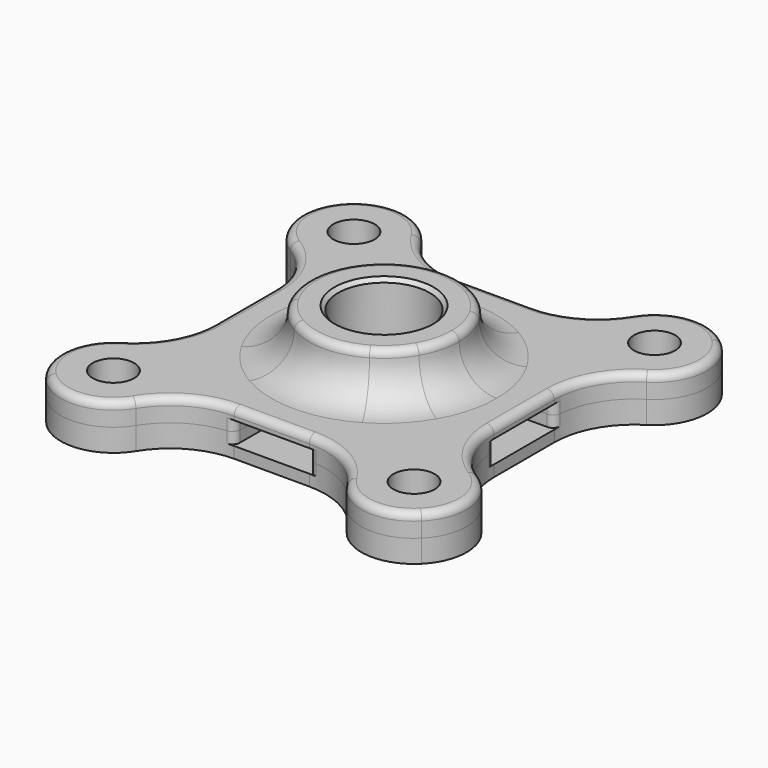
from build123d import *

# Parameters (mm, degrees)
F0_R           = 2.75
F0_R_2         = 9.25
F0_R_3         = 6.1
F1_DEPTH       = 3
F2_DEPTH       = 9
F3_DEPTH       = 1.5
F0_R_4         = 5
F4_DEPTH       = 3
F5_DEPTH       = 1.5
F6_SIZE        = 0.5
F7_R           = 5
F8_F1_R        = 0.9999
F8_F2_R        = 1
F8_2_T4_ANGLE  = 58.6491681138
F8_2_T10_ANGLE = 58.6491681138
F8_2_T16_ANGLE = 58.6491681138
F8_2_T22_ANGLE = 58.6491681138
F8_2_T25_DEPTH = 3.8925933322


# Not quite as in the source:
# - a fillet or chamfer that OpenCascade refuses, or shapes differently, is made with other operations: its cross-section is extruded or revolved along the edge and cut away or added
# - a fillet or chamfer is up to 0.001 mm smaller than in the source, because OpenCascade refuses the exact size
# - a feature names something its author has since deleted; it is built from what else it names


with BuildPart() as f1:
    # F0 (on Top) → F1 (new body)
    with BuildSketch(Plane.XY):
        with BuildLine():
            ThreePointArc((8.6602540378, 5), (9.6592582629, 2.588190451), (10, 0))
            ThreePointArc((10, 0), (9.6592582629, -2.588190451), (8.6602540378, -5))
            Line((8.6602540378, -5), (18.6602540378, -5))
            Line((18.6602540378, -5), (18.6602540378, 0))
            Line((18.6602540378, 0), (18.6602540378, 5))
            Line((18.6602540378, 5), (8.6602540378, 5))
        make_face()
        with BuildLine():
            ThreePointArc((5, 8.6602540378), (7.0710678119, 7.0710678119), (8.6602540378, 5))
            Line((8.6602540378, 5), (18.6602540378, 5))
            ThreePointArc((18.6602540378, 5), (20.0033649329, 10.1797503972), (23.6942299332, 14.0541892731))
            ThreePointArc((23.6942299332, 14.0541892731), (26.9539832777, 19.1986782332), (24.9497474683, 24.9497474683))
            ThreePointArc((24.9497474683, 24.9497474683), (19.1986782332, 26.9539832777), (14.0541892731, 23.6942299332))
            ThreePointArc((14.0541892731, 23.6942299332), (10.1797503972, 20.0033649329), (5, 18.6602540378))
            Line((5, 18.6602540378), (5, 8.6602540378))
        make_face()
        with Locations((20, 20)):
            Circle(F0_R, mode=Mode.SUBTRACT)
        with BuildLine():
            Line((18.6602540378, -5), (8.6602540378, -5))
            ThreePointArc((8.6602540378, -5), (7.0710678119, -7.0710678119), (5, -8.6602540378))
            Line((5, -8.6602540378), (5, -18.6602540378))
            ThreePointArc((5, -18.6602540378), (10.1797503972, -20.0033649329), (14.0541892731, -23.6942299332))
            ThreePointArc((14.0541892731, -23.6942299332), (19.1986782332, -26.9539832777), (24.9497474683, -24.9497474683))
            ThreePointArc((24.9497474683, -24.9497474683), (26.9539832777, -19.1986782332), (23.6942299332, -14.0541892731))
            ThreePointArc((23.6942299332, -14.0541892731), (20.0033649329, -10.1797503972), (18.6602540378, -5))
        make_face()
        with Locations((20, -20)):
            Circle(F0_R, mode=Mode.SUBTRACT)
        with BuildLine():
            ThreePointArc((-8.6602540378, 5), (-7.0710678119, 7.0710678119), (-5, 8.6602540378))
            Line((-5, 8.6602540378), (-5, 18.6602540378))
            ThreePointArc((-5, 18.6602540378), (-10.1797503972, 20.0033649329), (-14.0541892731, 23.6942299332))
            ThreePointArc((-14.0541892731, 23.6942299332), (-19.1986782332, 26.9539832777), (-24.9497474683, 24.9497474683))
            ThreePointArc((-24.9497474683, 24.9497474683), (-26.9539832777, 19.1986782332), (-23.6942299332, 14.0541892731))
            ThreePointArc((-23.6942299332, 14.0541892731), (-20.0033649329, 10.1797503972), (-18.6602540378, 5))
            Line((-18.6602540378, 5), (-8.6602540378, 5))
        make_face()
        with Locations((-20, 20)):
            Circle(F0_R, mode=Mode.SUBTRACT)
        with BuildLine():
            ThreePointArc((8.6602540378, -5), (9.6592582629, -2.588190451), (10, 0))
            ThreePointArc((10, 0), (9.6592582629, 2.588190451), (8.6602540378, 5))
            ThreePointArc((8.6602540378, 5), (7.0710678119, 7.0710678119), (5, 8.6602540378))
            ThreePointArc((5, 8.6602540378), (0, 10), (-5, 8.6602540378))
            ThreePointArc((-5, 8.6602540378), (-7.0710678119, 7.0710678119), (-8.6602540378, 5))
            ThreePointArc((-8.6602540378, 5), (-10, 0), (-8.6602540378, -5))
            ThreePointArc((-8.6602540378, -5), (-7.0710678119, -7.0710678119), (-5, -8.6602540378))
            ThreePointArc((-5, -8.6602540378), (0, -10), (5, -8.6602540378))
            ThreePointArc((5, -8.6602540378), (7.0710678119, -7.0710678119), (8.6602540378, -5))
        make_face()
        Circle(F0_R_2, mode=Mode.SUBTRACT)
        with BuildLine():
            Line((-5, -18.6602540378), (-5, -8.6602540378))
            ThreePointArc((-5, -8.6602540378), (-7.0710678119, -7.0710678119), (-8.6602540378, -5))
            Line((-8.6602540378, -5), (-18.6602540378, -5))
            ThreePointArc((-18.6602540378, -5), (-20.0033649329, -10.1797503972), (-23.6942299332, -14.0541892731))
            ThreePointArc((-23.6942299332, -14.0541892731), (-26.9539832777, -19.1986782332), (-24.9497474683, -24.9497474683))
            ThreePointArc((-24.9497474683, -24.9497474683), (-19.1986782332, -26.9539832777), (-14.0541892731, -23.6942299332))
            ThreePointArc((-14.0541892731, -23.6942299332), (-10.1797503972, -20.0033649329), (-5, -18.6602540378))
        make_face()
        with Locations((-20, -20)):
            Circle(F0_R, mode=Mode.SUBTRACT)
        with BuildLine():
            Line((5, -18.6602540378), (5, -8.6602540378))
            ThreePointArc((5, -8.6602540378), (0, -10), (-5, -8.6602540378))
            Line((-5, -8.6602540378), (-5, -18.6602540378))
            Line((-5, -18.6602540378), (0, -18.6602540378))
            Line((0, -18.6602540378), (5, -18.6602540378))
        make_face()
        Circle(F0_R_2)
        Circle(F0_R_3, mode=Mode.SUBTRACT)
        with BuildLine():
            ThreePointArc((-8.6602540378, -5), (-10, 0), (-8.6602540378, 5))
            Line((-8.6602540378, 5), (-18.6602540378, 5))
            Line((-18.6602540378, 5), (-18.6602540378, 0))
            Line((-18.6602540378, 0), (-18.6602540378, -5))
            Line((-18.6602540378, -5), (-8.6602540378, -5))
        make_face()
        with BuildLine():
            ThreePointArc((-5, 8.6602540378), (0, 10), (5, 8.6602540378))
            Line((5, 8.6602540378), (5, 18.6602540378))
            Line((5, 18.6602540378), (0, 18.6602540378))
            Line((0, 18.6602540378), (-5, 18.6602540378))
            Line((-5, 18.6602540378), (-5, 8.6602540378))
        make_face()
    extrude(amount=F1_DEPTH)

    # F0 (on Top) → F2 (join)
    with BuildSketch(Plane.XY):
        with BuildLine():
            ThreePointArc((8.6602540378, -5), (9.6592582629, -2.588190451), (10, 0))
            ThreePointArc((10, 0), (9.6592582629, 2.588190451), (8.6602540378, 5))
            ThreePointArc((8.6602540378, 5), (7.0710678119, 7.0710678119), (5, 8.6602540378))
            ThreePointArc((5, 8.6602540378), (0, 10), (-5, 8.6602540378))
            ThreePointArc((-5, 8.6602540378), (-7.0710678119, 7.0710678119), (-8.6602540378, 5))
            ThreePointArc((-8.6602540378, 5), (-10, 0), (-8.6602540378, -5))
            ThreePointArc((-8.6602540378, -5), (-7.0710678119, -7.0710678119), (-5, -8.6602540378))
            ThreePointArc((-5, -8.6602540378), (0, -10), (5, -8.6602540378))
            ThreePointArc((5, -8.6602540378), (7.0710678119, -7.0710678119), (8.6602540378, -5))
        make_face()
        Circle(F0_R_2, mode=Mode.SUBTRACT)
        Circle(F0_R_2)
        Circle(F0_R_3, mode=Mode.SUBTRACT)
    extrude(amount=F2_DEPTH)

    # F0 (on Top) → F3 (cut)
    with BuildSketch(Plane.XY):
        with BuildLine():
            ThreePointArc((8.6602540378, -5), (9.6592582629, -2.588190451), (10, 0))
            ThreePointArc((10, 0), (9.6592582629, 2.588190451), (8.6602540378, 5))
            ThreePointArc((8.6602540378, 5), (7.0710678119, 7.0710678119), (5, 8.6602540378))
            ThreePointArc((5, 8.6602540378), (0, 10), (-5, 8.6602540378))
            ThreePointArc((-5, 8.6602540378), (-7.0710678119, 7.0710678119), (-8.6602540378, 5))
            ThreePointArc((-8.6602540378, 5), (-10, 0), (-8.6602540378, -5))
            ThreePointArc((-8.6602540378, -5), (-7.0710678119, -7.0710678119), (-5, -8.6602540378))
            ThreePointArc((-5, -8.6602540378), (0, -10), (5, -8.6602540378))
            ThreePointArc((5, -8.6602540378), (7.0710678119, -7.0710678119), (8.6602540378, -5))
        make_face()
        Circle(F0_R_2, mode=Mode.SUBTRACT)
        Circle(F0_R_2)
        Circle(F0_R_3, mode=Mode.SUBTRACT)
        with BuildLine():
            Line((5, -18.6602540378), (5, -8.6602540378))
            ThreePointArc((5, -8.6602540378), (0, -10), (-5, -8.6602540378))
            Line((-5, -8.6602540378), (-5, -18.6602540378))
            Line((-5, -18.6602540378), (0, -18.6602540378))
            Line((0, -18.6602540378), (5, -18.6602540378))
        make_face()
        with BuildLine():
            ThreePointArc((-8.6602540378, -5), (-10, 0), (-8.6602540378, 5))
            Line((-8.6602540378, 5), (-18.6602540378, 5))
            Line((-18.6602540378, 5), (-18.6602540378, 0))
            Line((-18.6602540378, 0), (-18.6602540378, -5))
            Line((-18.6602540378, -5), (-8.6602540378, -5))
        make_face()
        with BuildLine():
            ThreePointArc((8.6602540378, 5), (9.6592582629, 2.588190451), (10, 0))
            ThreePointArc((10, 0), (9.6592582629, -2.588190451), (8.6602540378, -5))
            Line((8.6602540378, -5), (18.6602540378, -5))
            Line((18.6602540378, -5), (18.6602540378, 0))
            Line((18.6602540378, 0), (18.6602540378, 5))
            Line((18.6602540378, 5), (8.6602540378, 5))
        make_face()
        with BuildLine():
            ThreePointArc((-5, 8.6602540378), (0, 10), (5, 8.6602540378))
            Line((5, 8.6602540378), (5, 18.6602540378))
            Line((5, 18.6602540378), (0, 18.6602540378))
            Line((0, 18.6602540378), (-5, 18.6602540378))
            Line((-5, 18.6602540378), (-5, 8.6602540378))
        make_face()
    extrude(amount=F3_DEPTH, mode=Mode.SUBTRACT)

    # F6
    f6_edges = [f1.edges().sort_by_distance(p)[0] for p in [
        (-6.1, 0, 9),
    ]]
    chamfer(f6_edges, length=F6_SIZE)

    # F7
    f7_edges = [f1.edges().sort_by_distance(p)[0] for p in [
        (-8.660254, 5, 3),
    ]]
    fillet(f7_edges, radius=F7_R)

    # F8: fillet of radius 1 on 33 edges, made by hand

    # F8_f1 (radius 1 in the source; OpenCascade refuses exactly that, so slightly less here)
    f8_f1_edges = [f1.edges().sort_by_distance(p)[0] for p in [
        (18.6602540378, -5, 0.75),
        (18.6602540378, 5, 0.75),
        (5, 18.6602540378, 0.75),
        (-5, 18.6602540378, 0.75),
        (-18.6602540378, 5, 0.75),
        (-18.6602540378, -5, 0.75),
        (-5, -18.6602540378, 0.75),
        (5, -18.6602540378, 0.75),
        (-8.6602540378, 5, 9),
    ]]
    fillet(f8_f1_edges, radius=F8_F1_R)

    # F8_f2
    f8_f2_edges = [f1.edges().sort_by_distance(p)[0] for p in [
        (24.9497474683, 24.9497474683, 3),
        (-24.9497474683, 24.9497474683, 3),
        (-24.9497474683, -24.9497474683, 3),
        (24.9497474683, -24.9497474683, 3),
        (18.6602540378, 0, 3),
        (0, 18.6602540378, 3),
        (-18.6602540378, 0, 3),
        (0, -18.6602540378, 3),
        (20.0033649329, -10.1797503972, 3),
        (20.0033649329, 10.1797503972, 3),
        (10.1797503972, -20.0033649329, 3),
        (10.1797503972, 20.0033649329, 3),
        (-10.1797503972, -20.0033649329, 3),
        (-10.1797503972, 20.0033649329, 3),
        (-20.0033649329, -10.1797503972, 3),
        (-20.0033649329, 10.1797503972, 3),
    ]]
    fillet(f8_f2_edges, radius=F8_F2_R)


with BuildPart() as f4:
    # F0 (on Top) → F4 (new body)
    with BuildSketch(Plane.XY):
        with BuildLine():
            Line((-5, -18.6602540378), (-5, -8.6602540378))
            ThreePointArc((-5, -8.6602540378), (-7.0710678119, -7.0710678119), (-8.6602540378, -5))
            Line((-8.6602540378, -5), (-18.6602540378, -5))
            ThreePointArc((-18.6602540378, -5), (-20.0033649329, -10.1797503972), (-23.6942299332, -14.0541892731))
            ThreePointArc((-23.6942299332, -14.0541892731), (-26.9539832777, -19.1986782332), (-24.9497474683, -24.9497474683))
            ThreePointArc((-24.9497474683, -24.9497474683), (-19.1986782332, -26.9539832777), (-14.0541892731, -23.6942299332))
            ThreePointArc((-14.0541892731, -23.6942299332), (-10.1797503972, -20.0033649329), (-5, -18.6602540378))
        make_face()
        with Locations((-20, -20)):
            Circle(F0_R, mode=Mode.SUBTRACT)
        with BuildLine():
            Line((5, -18.6602540378), (5, -8.6602540378))
            ThreePointArc((5, -8.6602540378), (0, -10), (-5, -8.6602540378))
            Line((-5, -8.6602540378), (-5, -18.6602540378))
            Line((-5, -18.6602540378), (0, -18.6602540378))
            Line((0, -18.6602540378), (5, -18.6602540378))
        make_face()
        with BuildLine():
            Line((18.6602540378, -5), (8.6602540378, -5))
            ThreePointArc((8.6602540378, -5), (7.0710678119, -7.0710678119), (5, -8.6602540378))
            Line((5, -8.6602540378), (5, -18.6602540378))
            ThreePointArc((5, -18.6602540378), (10.1797503972, -20.0033649329), (14.0541892731, -23.6942299332))
            ThreePointArc((14.0541892731, -23.6942299332), (19.1986782332, -26.9539832777), (24.9497474683, -24.9497474683))
            ThreePointArc((24.9497474683, -24.9497474683), (26.9539832777, -19.1986782332), (23.6942299332, -14.0541892731))
            ThreePointArc((23.6942299332, -14.0541892731), (20.0033649329, -10.1797503972), (18.6602540378, -5))
        make_face()
        with Locations((20, -20)):
            Circle(F0_R, mode=Mode.SUBTRACT)
        with BuildLine():
            ThreePointArc((8.6602540378, 5), (9.6592582629, 2.588190451), (10, 0))
            ThreePointArc((10, 0), (9.6592582629, -2.588190451), (8.6602540378, -5))
            Line((8.6602540378, -5), (18.6602540378, -5))
            Line((18.6602540378, -5), (18.6602540378, 0))
            Line((18.6602540378, 0), (18.6602540378, 5))
            Line((18.6602540378, 5), (8.6602540378, 5))
        make_face()
        with BuildLine():
            ThreePointArc((5, 8.6602540378), (7.0710678119, 7.0710678119), (8.6602540378, 5))
            Line((8.6602540378, 5), (18.6602540378, 5))
            ThreePointArc((18.6602540378, 5), (20.0033649329, 10.1797503972), (23.6942299332, 14.0541892731))
            ThreePointArc((23.6942299332, 14.0541892731), (26.9539832777, 19.1986782332), (24.9497474683, 24.9497474683))
            ThreePointArc((24.9497474683, 24.9497474683), (19.1986782332, 26.9539832777), (14.0541892731, 23.6942299332))
            ThreePointArc((14.0541892731, 23.6942299332), (10.1797503972, 20.0033649329), (5, 18.6602540378))
            Line((5, 18.6602540378), (5, 8.6602540378))
        make_face()
        with Locations((20, 20)):
            Circle(F0_R, mode=Mode.SUBTRACT)
        with BuildLine():
            ThreePointArc((-5, 8.6602540378), (0, 10), (5, 8.6602540378))
            Line((5, 8.6602540378), (5, 18.6602540378))
            Line((5, 18.6602540378), (0, 18.6602540378))
            Line((0, 18.6602540378), (-5, 18.6602540378))
            Line((-5, 18.6602540378), (-5, 8.6602540378))
        make_face()
        with BuildLine():
            ThreePointArc((-8.6602540378, 5), (-7.0710678119, 7.0710678119), (-5, 8.6602540378))
            Line((-5, 8.6602540378), (-5, 18.6602540378))
            ThreePointArc((-5, 18.6602540378), (-10.1797503972, 20.0033649329), (-14.0541892731, 23.6942299332))
            ThreePointArc((-14.0541892731, 23.6942299332), (-19.1986782332, 26.9539832777), (-24.9497474683, 24.9497474683))
            ThreePointArc((-24.9497474683, 24.9497474683), (-26.9539832777, 19.1986782332), (-23.6942299332, 14.0541892731))
            ThreePointArc((-23.6942299332, 14.0541892731), (-20.0033649329, 10.1797503972), (-18.6602540378, 5))
            Line((-18.6602540378, 5), (-8.6602540378, 5))
        make_face()
        with Locations((-20, 20)):
            Circle(F0_R, mode=Mode.SUBTRACT)
        with BuildLine():
            ThreePointArc((-8.6602540378, -5), (-10, 0), (-8.6602540378, 5))
            Line((-8.6602540378, 5), (-18.6602540378, 5))
            Line((-18.6602540378, 5), (-18.6602540378, 0))
            Line((-18.6602540378, 0), (-18.6602540378, -5))
            Line((-18.6602540378, -5), (-8.6602540378, -5))
        make_face()
        with BuildLine():
            ThreePointArc((8.6602540378, -5), (9.6592582629, -2.588190451), (10, 0))
            ThreePointArc((10, 0), (9.6592582629, 2.588190451), (8.6602540378, 5))
            ThreePointArc((8.6602540378, 5), (7.0710678119, 7.0710678119), (5, 8.6602540378))
            ThreePointArc((5, 8.6602540378), (0, 10), (-5, 8.6602540378))
            ThreePointArc((-5, 8.6602540378), (-7.0710678119, 7.0710678119), (-8.6602540378, 5))
            ThreePointArc((-8.6602540378, 5), (-10, 0), (-8.6602540378, -5))
            ThreePointArc((-8.6602540378, -5), (-7.0710678119, -7.0710678119), (-5, -8.6602540378))
            ThreePointArc((-5, -8.6602540378), (0, -10), (5, -8.6602540378))
            ThreePointArc((5, -8.6602540378), (7.0710678119, -7.0710678119), (8.6602540378, -5))
        make_face()
        Circle(F0_R_2, mode=Mode.SUBTRACT)
        Circle(F0_R_2)
        Circle(F0_R_3, mode=Mode.SUBTRACT)
        Circle(F0_R_3)
        Circle(F0_R_4, mode=Mode.SUBTRACT)
        Circle(F0_R_4)
    extrude(amount=-F4_DEPTH)

    # F0 (on Top) → F5 (cut)
    with BuildSketch(Plane.XY):
        with BuildLine():
            ThreePointArc((-8.6602540378, -5), (-10, 0), (-8.6602540378, 5))
            Line((-8.6602540378, 5), (-18.6602540378, 5))
            Line((-18.6602540378, 5), (-18.6602540378, 0))
            Line((-18.6602540378, 0), (-18.6602540378, -5))
            Line((-18.6602540378, -5), (-8.6602540378, -5))
        make_face()
        with BuildLine():
            ThreePointArc((8.6602540378, -5), (9.6592582629, -2.588190451), (10, 0))
            ThreePointArc((10, 0), (9.6592582629, 2.588190451), (8.6602540378, 5))
            ThreePointArc((8.6602540378, 5), (7.0710678119, 7.0710678119), (5, 8.6602540378))
            ThreePointArc((5, 8.6602540378), (0, 10), (-5, 8.6602540378))
            ThreePointArc((-5, 8.6602540378), (-7.0710678119, 7.0710678119), (-8.6602540378, 5))
            ThreePointArc((-8.6602540378, 5), (-10, 0), (-8.6602540378, -5))
            ThreePointArc((-8.6602540378, -5), (-7.0710678119, -7.0710678119), (-5, -8.6602540378))
            ThreePointArc((-5, -8.6602540378), (0, -10), (5, -8.6602540378))
            ThreePointArc((5, -8.6602540378), (7.0710678119, -7.0710678119), (8.6602540378, -5))
        make_face()
        Circle(F0_R_2, mode=Mode.SUBTRACT)
        with BuildLine():
            ThreePointArc((-5, 8.6602540378), (0, 10), (5, 8.6602540378))
            Line((5, 8.6602540378), (5, 18.6602540378))
            Line((5, 18.6602540378), (0, 18.6602540378))
            Line((0, 18.6602540378), (-5, 18.6602540378))
            Line((-5, 18.6602540378), (-5, 8.6602540378))
        make_face()
        with BuildLine():
            ThreePointArc((8.6602540378, 5), (9.6592582629, 2.588190451), (10, 0))
            ThreePointArc((10, 0), (9.6592582629, -2.588190451), (8.6602540378, -5))
            Line((8.6602540378, -5), (18.6602540378, -5))
            Line((18.6602540378, -5), (18.6602540378, 0))
            Line((18.6602540378, 0), (18.6602540378, 5))
            Line((18.6602540378, 5), (8.6602540378, 5))
        make_face()
        with BuildLine():
            Line((5, -18.6602540378), (5, -8.6602540378))
            ThreePointArc((5, -8.6602540378), (0, -10), (-5, -8.6602540378))
            Line((-5, -8.6602540378), (-5, -18.6602540378))
            Line((-5, -18.6602540378), (0, -18.6602540378))
            Line((0, -18.6602540378), (5, -18.6602540378))
        make_face()
    extrude(amount=-F5_DEPTH, mode=Mode.SUBTRACT)

    # F8#2: fillet of radius 1 on 20 edges, made by hand


with BuildPart() as f8_2_tool2:
    # F8_2_s3 → F8_2_t4 (revolve)
    with BuildSketch(Plane(origin=(0, 0, 0), x_dir=(0, 0, 1), z_dir=(0.9628077651, 0.2701873563, 0))):
        with BuildLine():
            ThreePointArc((-1.5, -9), (-1.2071067812, -9.7071067812), (-0.5, -10))
            Line((-0.5, -10), (-1.5, -10))
            Line((-1.5, -10), (-1.5, -9))
        make_face()
    revolve(axis=Axis((0, 0, -1.5), (0, 0, 1)), revolution_arc=F8_2_T4_ANGLE)

    split(bisect_by=Plane.YZ.offset(-5), keep=Keep.BOTTOM)

    split(bisect_by=Plane.XZ.offset(-5), keep=Keep.BOTTOM)


with BuildPart() as f4_1:
    add(f4.part)

    # F8_2_t1: union F8_2_tool2
    add(f8_2_tool2.part)


with BuildPart() as f8_2_tool8:
    # F8_2_s9 → F8_2_t10 (revolve)
    with BuildSketch(Plane(origin=(0, 0, 0), x_dir=(0, 0, 1), z_dir=(-0.2701873563, 0.9628077651, 0))):
        with BuildLine():
            ThreePointArc((-0.5, -10), (-1.2071067812, -9.7071067812), (-1.5, -9))
            Line((-1.5, -9), (-1.5, -10))
            Line((-1.5, -10), (-0.5, -10))
        make_face()
    revolve(axis=Axis((0, 0, -1.5), (0, 0, 1)), revolution_arc=F8_2_T10_ANGLE)

    split(bisect_by=Plane.YZ.offset(-5), keep=Keep.BOTTOM)

    split(bisect_by=Plane.XZ.offset(5), keep=Keep.TOP)


with BuildPart() as f4_2:
    add(f4_1.part)

    # F8_2_t7: union F8_2_tool8
    add(f8_2_tool8.part)


with BuildPart() as f8_2_tool14:
    # F8_2_s15 → F8_2_t16 (revolve)
    with BuildSketch(Plane(origin=(0, 0, 0), x_dir=(0, 0, 1), z_dir=(-0.9628077651, -0.2701873563, 0))):
        with BuildLine():
            ThreePointArc((-1.5, -9), (-1.2071067812, -9.7071067812), (-0.5, -10))
            Line((-0.5, -10), (-1.5, -10))
            Line((-1.5, -10), (-1.5, -9))
        make_face()
    revolve(axis=Axis((0, 0, -1.5), (0, 0, 1)), revolution_arc=F8_2_T16_ANGLE)

    split(bisect_by=Plane.YZ.offset(5), keep=Keep.TOP)

    split(bisect_by=Plane.XZ.offset(5), keep=Keep.TOP)


with BuildPart() as f4_3:
    add(f4_2.part)

    # F8_2_t13: union F8_2_tool14
    add(f8_2_tool14.part)


with BuildPart() as f8_2_tool20:
    # F8_2_s21 → F8_2_t22 (revolve)
    with BuildSketch(Plane(origin=(0, 0, 0), x_dir=(0, 0, 1), z_dir=(0.2701873563, -0.9628077651, 0))):
        with BuildLine():
            ThreePointArc((-1.5, -9), (-1.2071067812, -9.7071067812), (-0.5, -10))
            Line((-0.5, -10), (-1.5, -10))
            Line((-1.5, -10), (-1.5, -9))
        make_face()
    revolve(axis=Axis((0, 0, -1.5), (0, 0, 1)), revolution_arc=F8_2_T22_ANGLE)

    split(bisect_by=Plane.XZ.offset(-5), keep=Keep.BOTTOM)

    split(bisect_by=Plane.YZ.offset(5), keep=Keep.TOP)


with BuildPart() as f4_4:
    add(f4_3.part)

    # F8_2_t19: union F8_2_tool20
    add(f8_2_tool20.part)

    # F8_2_s26 → F8_2_t25 (cut)
    with BuildSketch(Plane.XY.offset(-1.5)):
        with BuildLine():
            ThreePointArc((17.703216705, -5), (18.3793206074, -5.2631937072), (18.6995319248, -5.9142329738))
            ThreePointArc((18.6995319248, -5.9142329738), (18.6700780366, -5.4575381631), (18.6602540378, -5))
            Line((18.6602540378, -5), (17.703216705, -5))
        make_face()
        with BuildLine():
            ThreePointArc((17.703216705, 5), (18.3793206074, 5.2631937072), (18.6995319248, 5.9142329738))
            ThreePointArc((18.6995319248, 5.9142329738), (18.6700780366, 5.4575381631), (18.6602540378, 5))
            Line((18.6602540378, 5), (17.703216705, 5))
        make_face()
        with BuildLine():
            ThreePointArc((5, 17.703216705), (5.2631937072, 18.3793206074), (5.9142329738, 18.6995319248))
            ThreePointArc((5.9142329738, 18.6995319248), (5.4575381631, 18.6700780366), (5, 18.6602540378))
            Line((5, 18.6602540378), (5, 17.703216705))
        make_face()
        with BuildLine():
            ThreePointArc((-5, 17.703216705), (-5.2631937072, 18.3793206074), (-5.9142329738, 18.6995319248))
            ThreePointArc((-5.9142329738, 18.6995319248), (-5.4575381631, 18.6700780366), (-5, 18.6602540378))
            Line((-5, 18.6602540378), (-5, 17.703216705))
        make_face()
        with BuildLine():
            ThreePointArc((-17.703216705, 5), (-18.3793206074, 5.2631937072), (-18.6995319248, 5.9142329738))
            ThreePointArc((-18.6995319248, 5.9142329738), (-18.6700780366, 5.4575381631), (-18.6602540378, 5))
            Line((-18.6602540378, 5), (-17.703216705, 5))
        make_face()
        with BuildLine():
            ThreePointArc((-17.703216705, -5), (-18.3793206074, -5.2631937072), (-18.6995319248, -5.9142329738))
            ThreePointArc((-18.6995319248, -5.9142329738), (-18.6700780366, -5.4575381631), (-18.6602540378, -5))
            Line((-18.6602540378, -5), (-17.703216705, -5))
        make_face()
        with BuildLine():
            ThreePointArc((-5.9142329738, -18.6995319248), (-5.2631937072, -18.3793206074), (-5, -17.703216705))
            Line((-5, -17.703216705), (-5, -18.6602540378))
            ThreePointArc((-5, -18.6602540378), (-5.4575381631, -18.6700780366), (-5.9142329738, -18.6995319248))
        make_face()
        with BuildLine():
            ThreePointArc((5, -17.703216705), (5.2631937072, -18.3793206074), (5.9142329738, -18.6995319248))
            ThreePointArc((5.9142329738, -18.6995319248), (5.4575381631, -18.6700780366), (5, -18.6602540378))
            Line((5, -18.6602540378), (5, -17.703216705))
        make_face()
    extrude(amount=F8_2_T25_DEPTH, mode=Mode.SUBTRACT)


solid = Compound([f1.part, f4_4.part])
